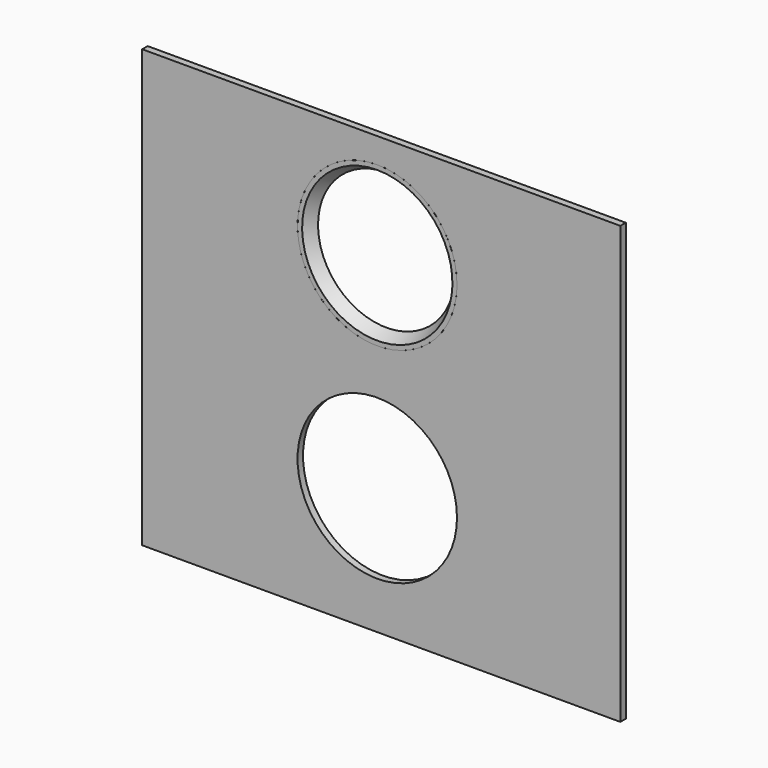
from build123d import *

# Parameters (mm, degrees)
F1_W     = 209.9018618464
F1_H     = 191.7395107448
F1_R     = 35
F2_DEPTH = 3
F5_W     = 80
F5_H     = 80
F5_R     = 1.5
F5_R_2   = 35
F6_DEPTH = 2


with BuildPart() as f2:
    # F1 (on offset) → F2 (new body)
    with BuildSketch(Plane.XZ.offset(5)):
        with Locations((1.7582438886, -49.7746858746)):
            Rectangle(F1_W, F1_H)
        with Locations((0, -90)):
            Circle(F1_R, mode=Mode.SUBTRACT)
        Circle(F1_R, mode=Mode.SUBTRACT)
    extrude(amount=-F2_DEPTH)


with BuildPart() as f4:
    # F3 (on Right) → F4 (revolve)
    with BuildSketch(Plane.YZ):
        Polygon((0, 35), (-5, 35), (-5, 33), (0, 30), align=None)
    revolve(axis=Axis((0, 1.602868408, 0), (0, -1, 0)))

    # F5 (on Front) → F6 (join)
    with BuildSketch(Plane.XZ):
        Rectangle(F5_W, F5_H)
        with Locations((-28, -28)):
            Circle(F5_R, mode=Mode.SUBTRACT)
        with Locations((28, -28)):
            Circle(F5_R, mode=Mode.SUBTRACT)
        with Locations((-28, 28)):
            Circle(F5_R, mode=Mode.SUBTRACT)
        Circle(F5_R_2, mode=Mode.SUBTRACT)
        with Locations((28, 28)):
            Circle(F5_R, mode=Mode.SUBTRACT)
    extrude(amount=F6_DEPTH)


solid = Compound([f2.part, f4.part])
